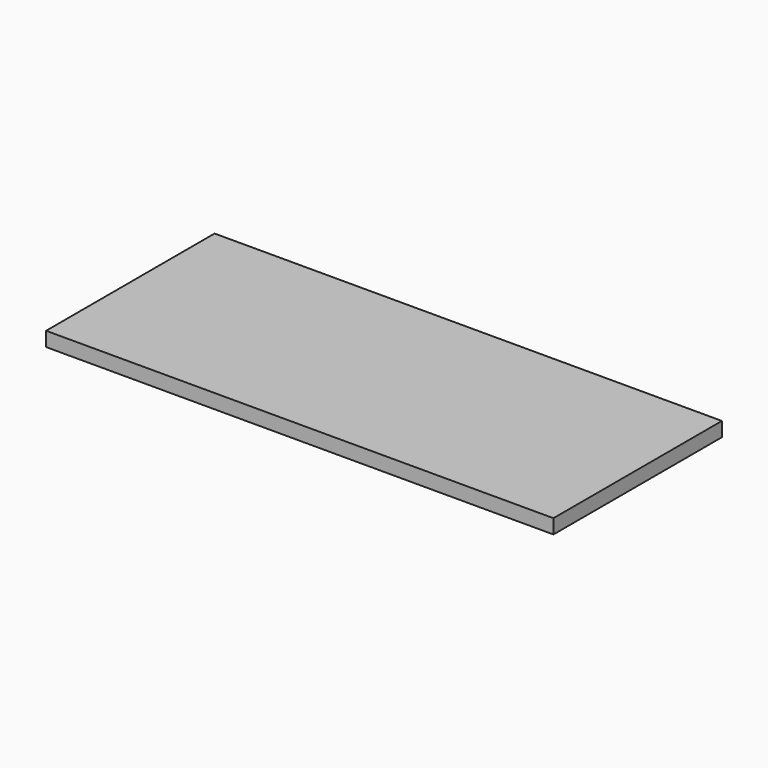
from build123d import *

# Parameters (mm, degrees)
F0_W     = 673.1
F0_H     = 279.4
F1_DEPTH = 19.05


# Not quite as in the source:
# - a length typed as a fraction of an inch, garbled in the dataset ("3 / 203.2 mm" for 3/8 in), is restored


with BuildPart() as f1:
    # F0 (on Top) → F1 (new body)
    with BuildSketch(Plane.XY):
        Rectangle(F0_W, F0_H)
    extrude(amount=F1_DEPTH)


solid = f1.part
